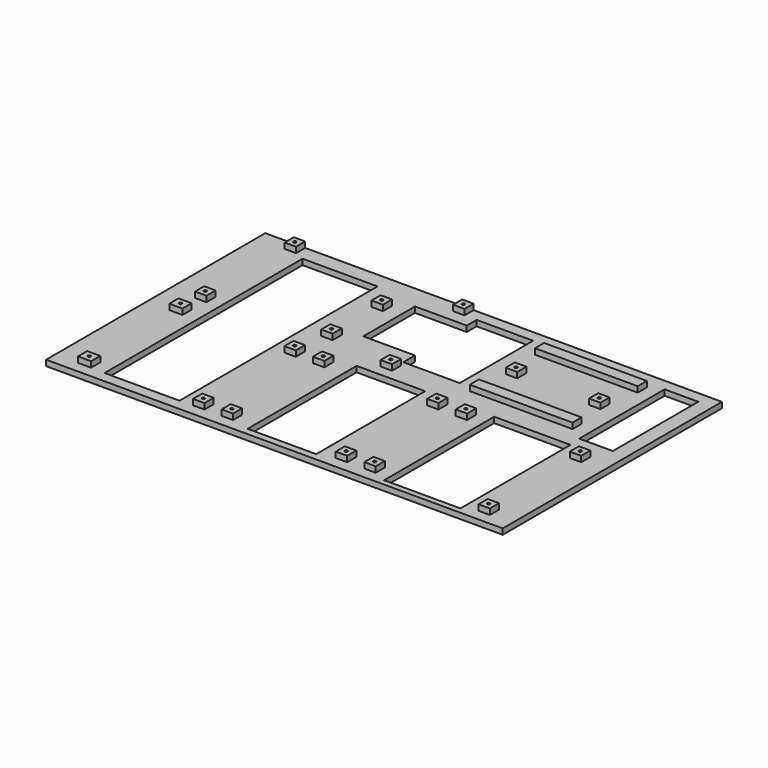
from build123d import *

# Parameters (mm, degrees)
F0_W     = 5.0798452705
F0_H     = 5.1181645604
F0_W_2   = 5.08
F0_H_2   = 5.08
F0_W_3   = 5.8267449073
F0_H_3   = 5.1171841682
F0_W_4   = 33.3881005645
F0_H_4   = 110.1423501968
F0_W_5   = 30.5098136887
F0_H_5   = 60.6358556543
F0_W_6   = 33.9637510478
F0_H_6   = 61.2115135882
F0_W_7   = 45.72
F0_W_8   = 14.9670690298
F0_H_7   = 47.5115125301
F1_DEPTH = 2.54
F2_DEPTH = 5.08
F5_D     = 1.27


# Not quite as in the source:
# - a feature of the source that left no trace in its solid (it failed there, or was rolled back) is left out
# - a feature names something its author has since deleted; it is built from what else it names


with BuildPart() as f1:
    # F0 (on Top) → F1 (new body)
    with BuildSketch(Plane.XY):
        Polygon((101.6, -60.96), (101.6, 60.96), (-8.89, 60.96), (-8.89, 55.88), (-13.97, 55.88), (-13.97, 60.96), (-83.82, 60.96), (-83.82, 55.88), (-88.9, 55.88), (-88.9, 60.96), (-101.6, 60.96), (-101.6, -60.96), align=None)
        Polygon((-91.44, -50.7502545385), (-85.6132550927, -50.7809177198), (-85.6132550927, -55.9297454615), (-91.44, -55.8990822802), align=None, mode=Mode.SUBTRACT)
        with Locations((-37.7266275464, -53.34)):
            Rectangle(F0_W, F0_H, mode=Mode.SUBTRACT)
        with Locations((-25.0266275464, -53.34)):
            Rectangle(F0_W_2, F0_H_2, mode=Mode.SUBTRACT)
        with Locations((-88.5266275464, -2.54)):
            Rectangle(F0_W_3, F0_H_3, mode=Mode.SUBTRACT)
        with Locations((-62.787938863, -1.0339058936)):
            Rectangle(F0_W_4, F0_H_4, mode=Mode.SUBTRACT)
        with Locations((-37.7266275464, -2.54)):
            Rectangle(F0_W_2, F0_H_2, mode=Mode.SUBTRACT)
        with Locations((-25.0266275464, -2.54)):
            Rectangle(F0_W_2, F0_H_2, mode=Mode.SUBTRACT)
        with Locations((25.7733724536, -53.34)):
            Rectangle(F0_W_2, F0_H_2, mode=Mode.SUBTRACT)
        with Locations((38.4733724536, -53.34)):
            Rectangle(F0_W_2, F0_H_2, mode=Mode.SUBTRACT)
        with Locations((89.2733724536, -53.34)):
            Rectangle(F0_W_2, F0_H_2, mode=Mode.SUBTRACT)
        with Locations((0.8221440949, -27.5141232414)):
            Rectangle(F0_W_5, F0_H_5, mode=Mode.SUBTRACT)
        with Locations((25.7733724536, -2.54)):
            Rectangle(F0_W_2, F0_H_2, mode=Mode.SUBTRACT)
        with Locations((38.4733724536, -2.54)):
            Rectangle(F0_W_2, F0_H_2, mode=Mode.SUBTRACT)
        with Locations((63.7606251985, -27.8019522084)):
            Rectangle(F0_W_6, F0_H_6, mode=Mode.SUBTRACT)
        with Locations((89.2733724536, -2.54)):
            Rectangle(F0_W_2, F0_H_2, mode=Mode.SUBTRACT)
        with Locations((-87.63, 10.16)):
            Rectangle(F0_W_2, F0_H_2, mode=Mode.SUBTRACT)
        with Locations((-5.08, 10.16)):
            Rectangle(F0_W_2, F0_H_2, mode=Mode.SUBTRACT)
        with Locations((-35.56, 15.24)):
            Rectangle(F0_W_2, F0_H_2, mode=Mode.SUBTRACT)
        with Locations((-35.56, 43.18)):
            Rectangle(F0_W_2, F0_H_2, mode=Mode.SUBTRACT)
        Polygon((-3.4952829592, 50.3914393485), (-3.4952829592, 55.88), (21.6417368501, 55.88), (21.6417368501, 15.0844864547), (-3.4952829592, 15.0844864547), (-3.4952829592, 21.6086003929), (-26.5215560794, 21.6086003929), (-26.5215560794, 50.3914393485), align=None, mode=Mode.SUBTRACT)
        with Locations((51.0222736127, 15.0563112164)):
            Rectangle(F0_W_7, F0_H_2, mode=Mode.SUBTRACT)
        with Locations((32.4802736127, 32.8363112164)):
            Rectangle(F0_W_2, F0_H_2, mode=Mode.SUBTRACT)
        with Locations((69.5642736127, 32.8363112164)):
            Rectangle(F0_W_2, F0_H_2, mode=Mode.SUBTRACT)
        with Locations((87.6503884792, 32.1242437349)):
            Rectangle(F0_W_8, F0_H_7, mode=Mode.SUBTRACT)
        with Locations((51.5818764424, 50.6163112164)):
            Rectangle(F0_W_7, F0_H_2, mode=Mode.SUBTRACT)
    extrude(amount=F1_DEPTH)

    # F0 (on Top) → F2 (join)
    with BuildSketch(Plane.XY):
        with Locations((-86.36, 58.42)):
            Rectangle(F0_W_2, F0_H_2)
        with Locations((-35.56, 43.18)):
            Rectangle(F0_W_2, F0_H_2)
        with Locations((-11.43, 58.42)):
            Rectangle(F0_W_2, F0_H_2)
        with Locations((-35.56, 15.24)):
            Rectangle(F0_W_2, F0_H_2)
        with Locations((-5.08, 10.16)):
            Rectangle(F0_W_2, F0_H_2)
        with Locations((-87.63, 10.16)):
            Rectangle(F0_W_2, F0_H_2)
        with Locations((-88.5266275464, -2.54)):
            Rectangle(F0_W_3, F0_H_3)
        with Locations((-37.7266275464, -2.54)):
            Rectangle(F0_W_2, F0_H_2)
        with Locations((-37.7266275464, -53.34)):
            Rectangle(F0_W, F0_H)
        with Locations((-25.0266275464, -2.54)):
            Rectangle(F0_W_2, F0_H_2)
        with Locations((25.7733724536, -2.54)):
            Rectangle(F0_W_2, F0_H_2)
        with Locations((38.4733724536, -2.54)):
            Rectangle(F0_W_2, F0_H_2)
        with Locations((89.2733724536, -2.54)):
            Rectangle(F0_W_2, F0_H_2)
        with Locations((89.2733724536, -53.34)):
            Rectangle(F0_W_2, F0_H_2)
        with Locations((38.4733724536, -53.34)):
            Rectangle(F0_W_2, F0_H_2)
        with Locations((25.7733724536, -53.34)):
            Rectangle(F0_W_2, F0_H_2)
        with Locations((-25.0266275464, -53.34)):
            Rectangle(F0_W_2, F0_H_2)
        Polygon((-85.6132550927, -55.9297454615), (-85.6132550927, -50.7809177198), (-91.44, -50.7502545385), (-91.44, -55.8990822802), align=None)
        with Locations((32.4802736127, 32.8363112164)):
            Rectangle(F0_W_2, F0_H_2)
        with Locations((51.0222736127, 15.0563112164)):
            Rectangle(F0_W_7, F0_H_2)
        with Locations((69.5642736127, 32.8363112164)):
            Rectangle(F0_W_2, F0_H_2)
        with Locations((51.5818764424, 50.6163112164)):
            Rectangle(F0_W_7, F0_H_2)
    extrude(amount=F2_DEPTH)

    # F5 (through all)
    with Locations(Plane(origin=(0, 0, 0), x_dir=(1, 0, 0), z_dir=(0, 0, -1))):
        with Locations((-25.0266275464, 2.54), (-37.7266275464, 2.54), (25.7733724536, 2.54), (38.4733724536, 2.54), (89.2733724536, 2.54), (89.2733724536, 53.34), (38.4733724536, 53.34), (25.7733724536, 53.34), (-25.0266275464, 53.34), (-37.7266275464, 53.34), (-88.5266275464, 53.34), (-88.5266275464, 2.54), (-87.63, -10.16), (-35.56, -15.24), (-5.08, -10.16), (32.4802736127, -32.8363112164), (69.5642736127, -32.8363112164), (-11.43, -58.42), (-35.56, -43.18), (-86.36, -58.42)):
            Hole(F5_D / 2)


solid = f1.part
